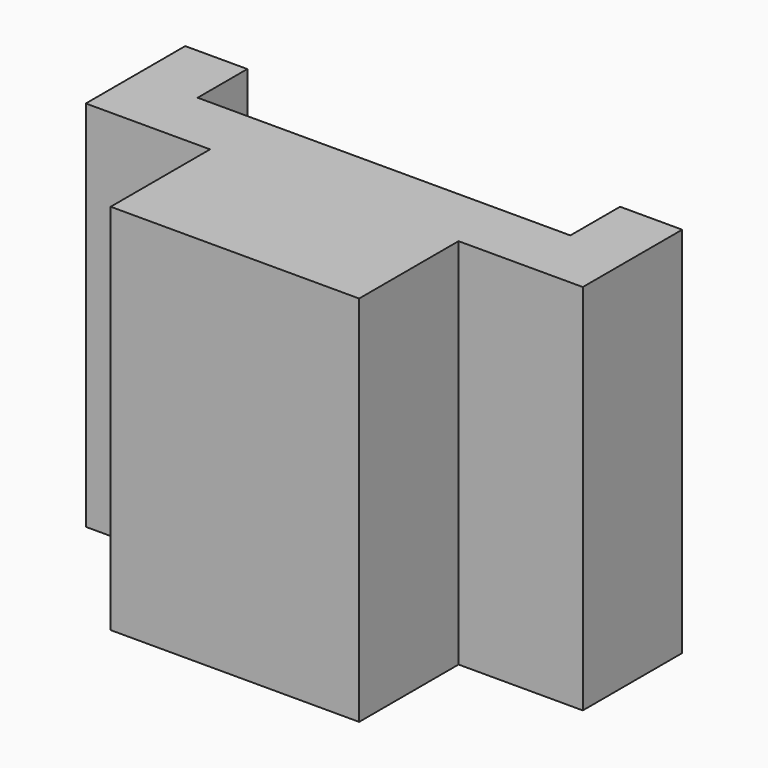
from build123d import *

# Parameters (mm, degrees)
F0_W     = 10
F0_H     = 60
F1_DEPTH = 40
F2_W     = 20
F2_H     = 60
F3_DEPTH = 20
F4_DEPTH = 10


with BuildPart() as f1:
    # F0 (on Front) → F1 (new body)
    with BuildSketch(Plane.XZ):
        with Locations((-75, -30)):
            Rectangle(F0_W, F0_H)
        with Locations((-65, -30)):
            Rectangle(F0_W, F0_H)
        Polygon((-20, 0), (-60, 0), (-60, -60), (-21.7804121599, -60), (-20, -60), align=None)
        with Locations((-15, -30)):
            Rectangle(F0_W, F0_H)
        with Locations((-5, -30)):
            Rectangle(F0_W, F0_H)
    extrude(amount=F1_DEPTH)

    # F0 (on Front) + F2 (on face) → F3 (cut)
    with BuildSketch(Plane.XZ):
        with Locations((-75, -30)):
            Rectangle(F0_W, F0_H)
        with Locations((-65, -30)):
            Rectangle(F0_W, F0_H)
        Polygon((-20, 0), (-60, 0), (-60, -60), (-21.7804121599, -60), (-20, -60), align=None)
        with Locations((-15, -30)):
            Rectangle(F0_W, F0_H)
        with Locations((-5, -30)):
            Rectangle(F0_W, F0_H)
    with BuildSketch(Plane.XZ.offset(40)):
        with Locations((-70, -30)):
            Rectangle(F2_W, F2_H)
        with Locations((-10, -30)):
            Rectangle(F2_W, F2_H)
    extrude(amount=-F3_DEPTH, mode=Mode.SUBTRACT)

    # F0 (on Front) → F4 (cut)
    with BuildSketch(Plane.XZ):
        with Locations((-65, -30)):
            Rectangle(F0_W, F0_H)
        Polygon((-20, 0), (-60, 0), (-60, -60), (-21.7804121599, -60), (-20, -60), align=None)
        with Locations((-15, -30)):
            Rectangle(F0_W, F0_H)
    extrude(amount=F4_DEPTH, mode=Mode.SUBTRACT)


solid = f1.part
